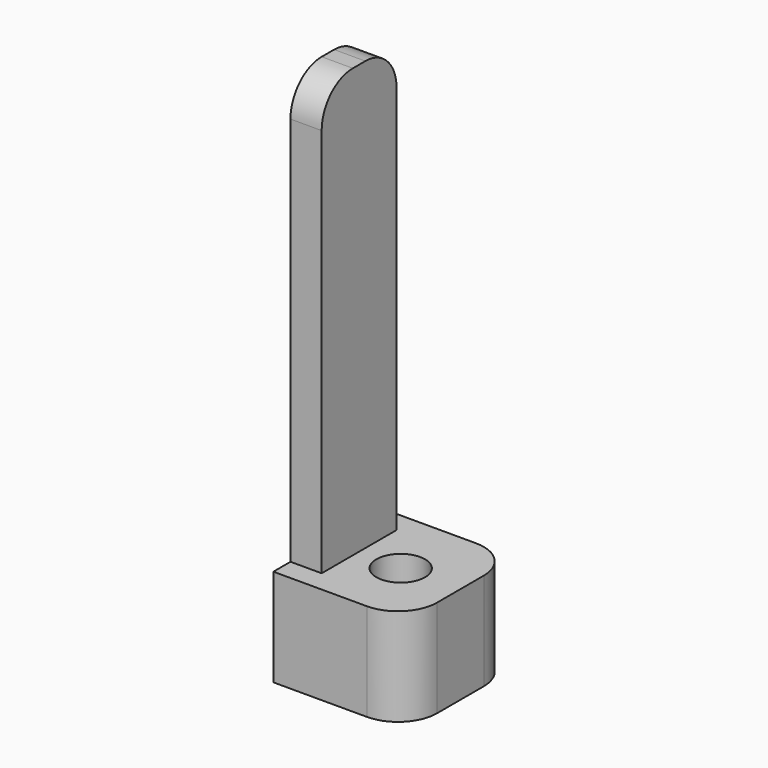
from build123d import *

# Parameters (mm, degrees)
F1_DEPTH  = 5
F2_R      = 2.5
F3_DEPTH  = 1.6
F4_R      = 1.25
F5_DEPTH  = 3.4
F6_W      = 2
F6_H      = 4.8
F7_DEPTH  = 22
F8_R      = 2
F9_DEPTH  = 0.2
F10_DEPTH = 0.2


# Not quite as in the source:
# - a feature names something its author has since deleted; it is built from what else it names


with BuildPart() as f1:
    # F0 (on Top) → F1 (new body)
    with BuildSketch(Plane.XY):
        with BuildLine():
            Line((1, 21.8148477226), (-4, 21.8148477226))
            Line((-4, 21.8148477226), (-4, 14.8148477226))
            Line((-4, 14.8148477226), (1, 14.8148477226))
            ThreePointArc((1, 14.8148477226), (2.4142135624, 15.4006341603), (3, 16.8148477226))
            Line((3, 16.8148477226), (3, 19.8148477226))
            ThreePointArc((3, 19.8148477226), (2.4142135624, 21.229061285), (1, 21.8148477226))
        make_face()
    extrude(amount=F1_DEPTH)

    # F2 (on face) → F3 (cut)
    with BuildSketch(Plane(origin=(0, 0, 0), x_dir=(1, 0, 0), z_dir=(0, 0, -1))):
        with Locations((0, -18.2346012443)):
            Circle(F2_R)
    extrude(amount=-F3_DEPTH, mode=Mode.SUBTRACT)

    # F4 (on face) → F5 (cut)
    with BuildSketch(Plane(origin=(0, 0, 1.6), x_dir=(1, 0, 0), z_dir=(0, 0, -1))):
        with Locations((0, -18.2346012443)):
            Circle(F4_R)
    extrude(amount=-F5_DEPTH, mode=Mode.SUBTRACT)

    # F6 (on face) → F7 (join)
    with BuildSketch(Plane.XY.offset(5)):
        with Locations((-3, 18.3148477226)):
            Rectangle(F6_W, F6_H)
    extrude(amount=F7_DEPTH)

    # F8
    f8_edges = [f1.edges().sort_by_distance(p)[0] for p in [
        (-3, 20.714848, 27),
        (-3, 15.914848, 27),
    ]]
    fillet(f8_edges, radius=F8_R)

    # F9 (cut): a face of the model
    f9_faces = [f1.faces().sort_by_distance(p)[0] for p in [
        (-2, 18.3148477226, 15.8255925745),
    ]]
    extrude(f9_faces, amount=-F9_DEPTH, mode=Mode.SUBTRACT)

    # F10 (cut): a face of the model
    f10_faces = [f1.faces().sort_by_distance(p)[0] for p in [
        (-4, 18.3148477226, 12.4674053391),
    ]]
    extrude(f10_faces, amount=-F10_DEPTH, mode=Mode.SUBTRACT)


solid = f1.part
